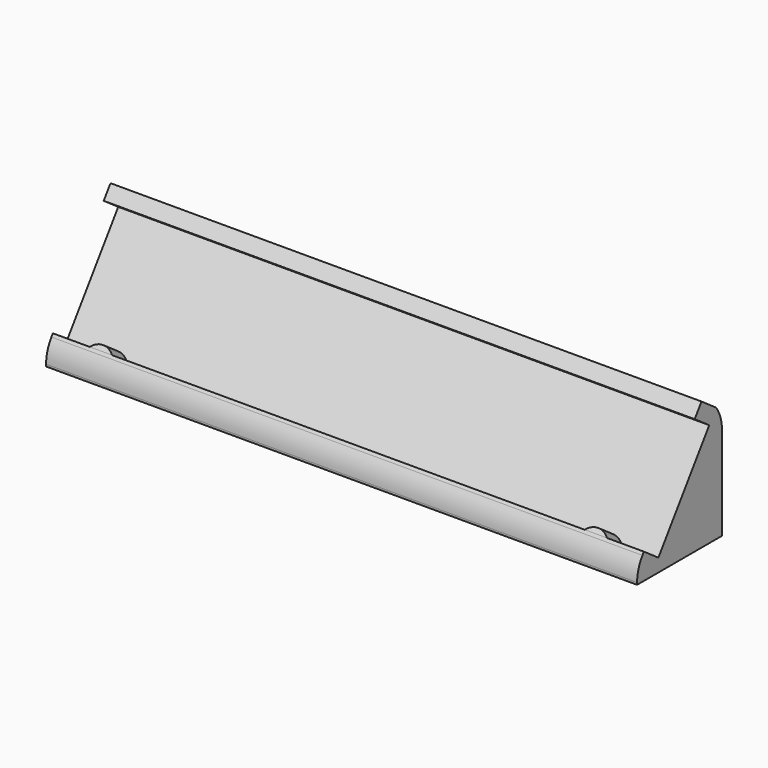
from build123d import *

# Parameters (mm, degrees)
F1_DEPTH    = 40
F2_R        = 5
F3_T1_DEPTH = 95
F5_DEPTH    = 3


# Not quite as in the source:
# - a fillet or chamfer that OpenCascade refuses, or shapes differently, is made with other operations: its cross-section is extruded or revolved along the edge and cut away or added


with BuildPart() as f1:
    # F0 (on Right) → F1 (new body, symmetric)
    with BuildSketch(Plane.YZ):
        Polygon((0.0953060592, 0.1361111585), (0, 0), (11.9932583499, 0), (11.9932583499, 15.7), (10.9932583499, 15.7), (9.8461054772, 14.0616959114), (1.2424589319, 1.7744152471), align=None)
        Polygon((7.3886493443, 15.7824252205), (9.8461054772, 14.0616959114), (10.9932583499, 15.7), (8.535802217, 17.4207293091), align=None)
        Polygon((-2.3621500736, 1.8568404676), (0.0953060592, 0.1361111585), (1.2424589319, 1.7744152471), (-1.2149972009, 3.4951445561), align=None)
        Polygon((-2.3621500736, 0), (0, 0), (0.0953060592, 0.1361111585), (-2.3621500736, 1.8568404676), align=None)
    extrude(amount=F1_DEPTH, both=True)

    # F2
    f2_edges = [f1.edges().sort_by_distance(p)[0] for p in [
        (0, -2.36215, 1.85684),
    ]]
    fillet(f2_edges, radius=F2_R)

    # F3: fillet of radius 5 on 1 edges, made by hand

    # F3_s2 → F3_t1 (cut)
    with BuildSketch(Plane.YZ.offset(-47.5)):
        with BuildLine():
            ThreePointArc((11.9932583499, 12.7), (11.7366748401, 14.2811388301), (10.9932583499, 15.7))
            Line((10.9932583499, 15.7), (11.9932583499, 15.7))
            Line((11.9932583499, 15.7), (11.9932583499, 12.7))
        make_face()
    extrude(amount=F3_T1_DEPTH, mode=Mode.SUBTRACT)

    # F4 (on face) → F5 (join)
    with BuildSketch(Plane(origin=(0, 0, 0), x_dir=(1, 0, 0), z_dir=(0, -0.8191520443, 0.5735764364))):
        with BuildLine():
            Line((-35, 2.1661610436), (-32, 2.1661610436))
            ThreePointArc((-32, 2.1661610436), (-33.5, 2.843285388), (-35, 2.1661610436))
        make_face()
        with BuildLine():
            ThreePointArc((35, 2.1661610436), (33.5, 2.843285388), (32, 2.1661610436))
            Line((32, 2.1661610436), (35, 2.1661610436))
        make_face()
    extrude(amount=F5_DEPTH)


solid = f1.part
